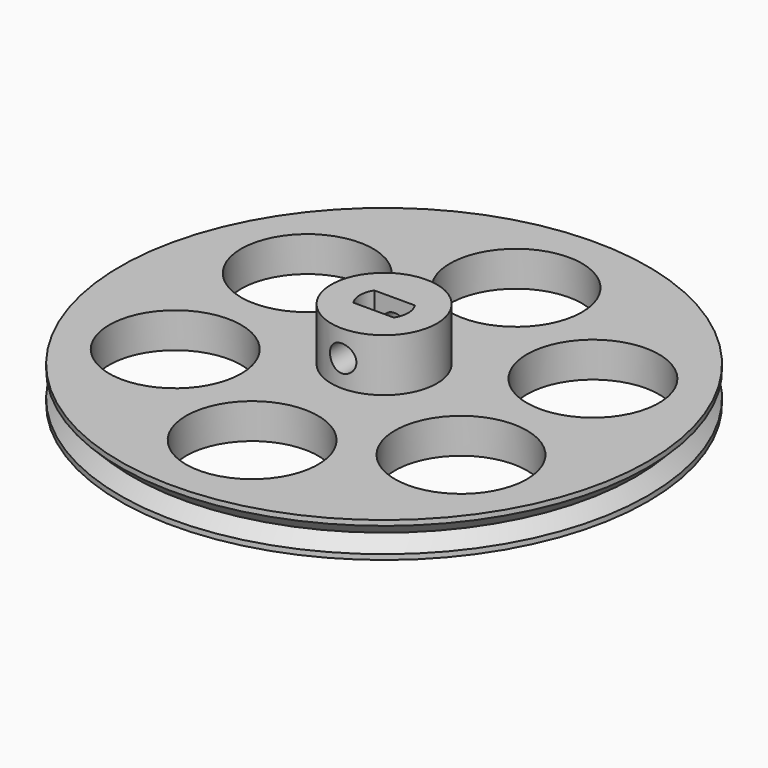
from build123d import *

# Parameters (mm, degrees)
F0_R             = 30
F0_R_2           = 6
F1_DEPTH         = 4
F2_DEPTH         = 6
F3_R             = 1.5
F4_DEPTH         = 12.5
F5_W             = 4.6
F5_H             = 3
F6_DEPTH         = 9.4
F9_R             = 7.5
F10_DEPTH        = 25
F10_COPIES_COUNT = 6


# Not quite as in the source:
# - a pattern or mirror of a feature is missing from the dataset's text; its kind, count and spacing are read off the source's solid


with BuildPart() as f1:
    # F0 (on Top) → F1 (new body)
    with BuildSketch(Plane.XY):
        Circle(F0_R)
        Circle(F0_R_2, mode=Mode.SUBTRACT)
        Circle(F0_R_2)
    extrude(amount=-F1_DEPTH)

    # F0 (on Top) → F2 (join)
    with BuildSketch(Plane.XY):
        Circle(F0_R_2)
    extrude(amount=F2_DEPTH)

    # F3 (on Front) → F4 (cut, symmetric)
    with BuildSketch(Plane.XZ):
        with Locations((0, 3)):
            Circle(F3_R)
    extrude(amount=F4_DEPTH, both=True, mode=Mode.SUBTRACT)

    # F5 (on face) → F6 (cut)
    with BuildSketch(Plane.XY.offset(6)):
        Rectangle(F5_W, F5_H)
        with BuildLine():
            ThreePointArc((-2.3, 1.5), (-2.7459060435, 0), (-2.3, -1.5))
            Line((-2.3, -1.5), (-2.3, 1.5))
        make_face()
        with BuildLine():
            Line((2.3, 1.5), (2.3, -1.5))
            ThreePointArc((2.3, -1.5), (2.745183651, 0), (2.3, 1.5))
        make_face()
    extrude(amount=-F6_DEPTH, mode=Mode.SUBTRACT)

    # F7 (on Front) → F8 (revolve, cut)
    with BuildSketch(Plane.XZ):
        Polygon((30, -3.4142135624), (30, -0.5857864376), (28.5857864376, -2), align=None)
    revolve(axis=Axis((0, 0, 0.7614716887), (0, 0, -1)), mode=Mode.SUBTRACT)

    # F9 (on face) → F10 (cut)
    with BuildSketch(Plane.XY):
        with Locations((0, 18.75)):
            Circle(F9_R)
    f10 = extrude(amount=-F10_DEPTH, mode=Mode.SUBTRACT)

    # F10_copies: F10 ×6 about axis
    f10_copies_axis = Axis((0, 0, 0), (0, 0, 1))
    for i in range(1, F10_COPIES_COUNT):
        add(f10.rotate(f10_copies_axis, i * 360 / F10_COPIES_COUNT), mode=Mode.SUBTRACT)


solid = f1.part
